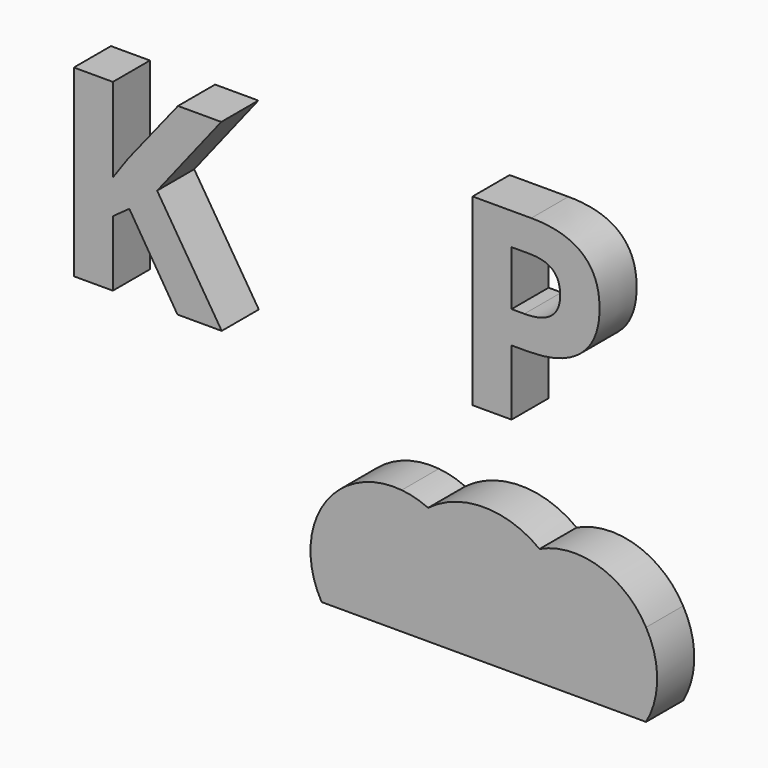
from build123d import *

# Parameters (mm, degrees)
F0_TEXT_SIZE = 35.2777777778
F1_DEPTH     = 6.35


# Not quite as in the source:
# - the program builds the solid bodies; features that only make, move or delete a surface that nothing else refers to are left out
# - Text() gives the source's letters only with a copy of the font that has no kerning and outlines rounded to 1/6400 em; it was checked with that copy


with BuildPart() as f1:
    # F0 (on Front) → F1 (new body)
    with BuildSketch(Plane.XZ):
        with BuildLine():
            ThreePointArc((-22.225, 11.4060379189), (-23.7506451088, 5.7030189594), (-22.225, 0))
            Line((-22.225, 0), (22.225, 0))
            ThreePointArc((22.225, 0), (23.7506451088, 5.7030189594), (22.225, 11.4060379189))
            ThreePointArc((22.225, 11.4060379189), (15.8597637653, 16.6455821123), (7.6325169088, 16.1150495111))
            ThreePointArc((7.6325169088, 16.1150495111), (0, 18.6793906953), (-7.6325169088, 16.1150495111))
            ThreePointArc((-7.6325169088, 16.1150495111), (-9.3996822705, 16.7431714436), (-11.2458134759, 17.0736410335))
            ThreePointArc((-11.2458134759, 17.0736410335), (-17.5679084489, 15.8525479494), (-22.225, 11.4060379189))
        make_face()
        with Locations((-4.7125581765, 30.4649711311)):
            Text('P', F0_TEXT_SIZE, font='Open Sans', font_style=FontStyle.BOLD, text_align=(TextAlign.LEFT, TextAlign.BOTTOM))
        with Locations((-59.3350535664, 28.2556206644)):
            Text('K', F0_TEXT_SIZE, font='Open Sans', font_style=FontStyle.BOLD, text_align=(TextAlign.LEFT, TextAlign.BOTTOM))
    extrude(amount=F1_DEPTH)


solid = f1.part
